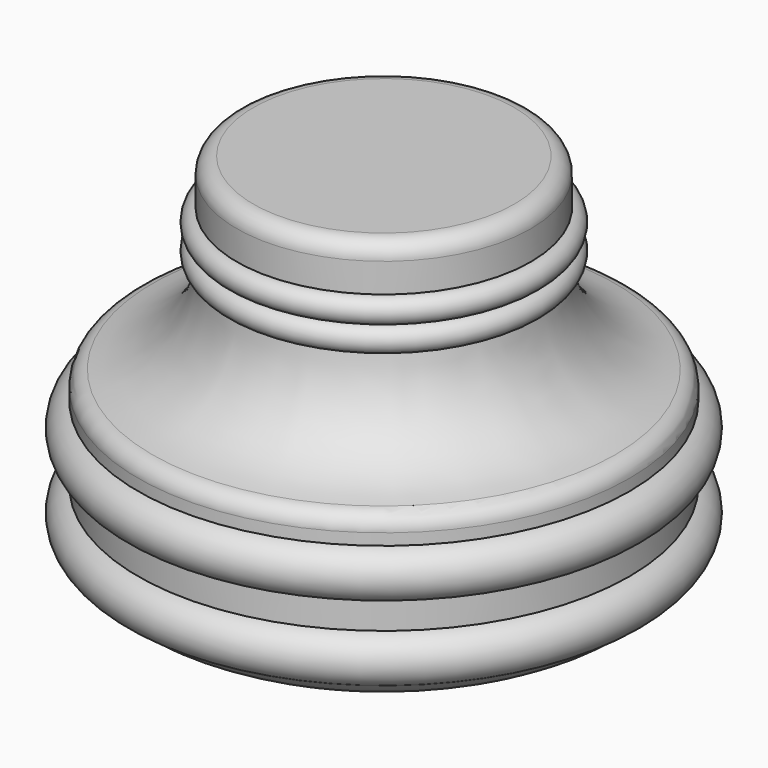
from build123d import *

# Parameters (mm, degrees)
F3_R = 1
F5_R = 1


# Not quite as in the source:
# - a fillet or chamfer that OpenCascade refuses, or shapes differently, is made with other operations: its cross-section is extruded or revolved along the edge and cut away or added


with BuildPart() as f1:
    # F0 (on Front) → F1 (revolve)
    with BuildSketch(Plane.XZ):
        with BuildLine():
            Line((-54.8627413809, 43.9864732325), (-63.8383940968, 43.9864732325))
            Line((-63.8383940968, 43.9864732325), (-63.8383940968, 21.686617285))
            Line((-63.8383940968, 21.686617285), (-48.8383940968, 21.686617285))
            Line((-48.8383940968, 21.686617285), (-48.8383940968, 23.3574478392))
            ThreePointArc((-48.8383940968, 23.3574478392), (-47.7196917759, 24.8081759598), (-48.8383940968, 26.2589040804))
            Line((-48.8383940968, 26.2589040804), (-48.8383940968, 27.9297346346))
            ThreePointArc((-48.8383940968, 27.9297346346), (-47.7196917759, 29.3804627552), (-48.8383940968, 30.8311908759))
            Line((-48.8383940968, 30.8311908759), (-48.8383940968, 32.5317010283))
            Line((-48.8383940968, 32.5317010283), (-54.8627413809, 32.5317010283))
            Line((-54.8627413809, 32.5317010283), (-54.8627413809, 38.1189764225))
            ThreePointArc((-54.8627413809, 38.1189764225), (-54.1422003229, 38.8903204691), (-54.8627413809, 39.6616645157))
            ThreePointArc((-54.8627413809, 39.6616645157), (-54.1422003229, 40.4330085623), (-54.8627413809, 41.2043526089))
            Line((-54.8627413809, 41.2043526089), (-54.8627413809, 43.9864732325))
        make_face()
    revolve(axis=Axis((-63.8383940968, 0, 32.8365452588), (0, 0, -1)))

    # F2: fillet of radius 5 on 1 edges, made by hand

    # F2_s1 → F2_t2 (revolve, cut)
    with BuildSketch(Plane.XZ):
        with BuildLine():
            ThreePointArc((-52.5688941707, 21.686617285), (-50.525104459, 22.1234031092), (-48.8383940968, 23.3574478392))
            Line((-48.8383940968, 23.3574478392), (-48.8383940968, 21.686617285))
            Line((-48.8383940968, 21.686617285), (-52.5688941707, 21.686617285))
        make_face()
    revolve(axis=Axis((-63.8383940968, 0, 21.686617285), (0, 0, -1)), mode=Mode.SUBTRACT)

    # F3
    f3_edges = [f1.edges().sort_by_distance(p)[0] for p in [
        (-78.838394, 0, 32.531701),
    ]]
    fillet(f3_edges, radius=F3_R)

    # F4: fillet of radius 6 on 1 edges, made by hand

    # F4_s1 → F4_t2 (revolve)
    with BuildSketch(Plane.XZ):
        with BuildLine():
            ThreePointArc((-49.7004398219, 32.5221396272), (-53.2831091702, 34.39679679), (-54.8627413809, 38.1189764225))
            Line((-54.8627413809, 38.1189764225), (-55.4617441018, 38.0843969428))
            ThreePointArc((-55.4617441018, 38.0843969428), (-55.4627413809, 35.3253387254), (-55.4627413809, 32.5317010283))
            Line((-55.4627413809, 32.5317010283), (-54.8627413809, 31.9317010283))
            ThreePointArc((-54.8627413809, 31.9317010283), (-49.8383940968, 31.9317010283), (-49.7832123868, 31.9278764679))
            Line((-49.7832123868, 31.9278764679), (-49.7004398219, 32.5221396272))
        make_face()
    revolve(axis=Axis((-63.8383940968, 0, 32.5317010283), (0, 0, -1)))

    # F5
    f5_edges = [f1.edges().sort_by_distance(p)[0] for p in [
        (-72.814047, 0, 43.986473),
    ]]
    fillet(f5_edges, radius=F5_R)


solid = f1.part
